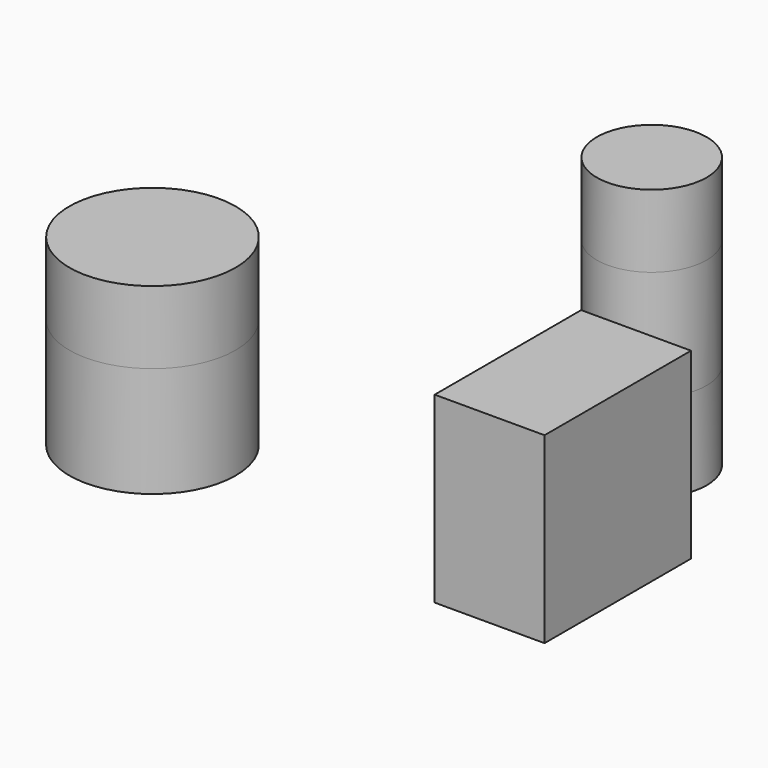
from build123d import *

# Parameters (mm, degrees)
F0_W        = 15
F0_H        = 25
F3_DEPTH    = 25
F2_R        = 7.5
F4_DEPTH    = 25
F2_R_2      = 11.3476620201
F4_FACE_R   = 11.3476620201
F4_FACE_R_2 = 7.5
F4_FACE1_R  = 7.5
F5_DEPTH    = 12
F6_DEPTH    = 15.07007


# Not quite as in the source:
# - the program builds the solid bodies; features that only make, move or delete a surface that nothing else refers to are left out


with BuildPart() as f3:
    # F0 (on Top) → F3 (new body)
    with BuildSketch(Plane.XY):
        with Locations((37.4109183252, -27.5365926325)):
            Rectangle(F0_W, F0_H)
    extrude(amount=F3_DEPTH)


with BuildPart() as f4:
    # F2 (on Top) → F4 (new body)
    with BuildSketch(Plane.XY):
        with Locations((13.7380197997, 17.2195071473)):
            Circle(F2_R)
    extrude(amount=F4_DEPTH)


with BuildPart() as f4b:
    # F2 (on Top) → F4, piece 2 (new body)
    with BuildSketch(Plane.XY):
        with Locations((-16.3307688936, -30.4005464111)):
            Circle(F2_R_2)
    extrude(amount=F4_DEPTH)

    # F4_face (on face) + F4_face1 (on face) → F5 (join)
    with BuildSketch(Plane(origin=(-16.3307688936, -30.4005464111, 25), x_dir=(1, 0, 0), z_dir=(0, 0, 1))):
        Circle(F4_FACE_R)
        with Locations((30.0687886933, 47.6200535584)):
            Circle(F4_FACE_R_2)
    with BuildSketch(Plane(origin=(13.7380197997, 17.2195071473, 0), x_dir=(1, 0, 0), z_dir=(0, 0, -1))):
        Circle(F4_FACE1_R)
    extrude(amount=-F5_DEPTH, dir=(0, 0, 1))


with BuildPart() as f6:
    # F2 (on Top) → F6 (new body)
    with BuildSketch(Plane.XY):
        with Locations((13.7380197997, 17.2195071473)):
            Circle(F2_R)
    extrude(amount=F6_DEPTH)


with BuildPart() as f6b:
    # F2 (on Top) → F6, piece 2 (new body)
    with BuildSketch(Plane.XY):
        with Locations((-16.3307688936, -30.4005464111)):
            Circle(F2_R_2)
    extrude(amount=F6_DEPTH)


solid = Compound([f3.part, f4.part, f4b.part, f6.part, f6b.part])
